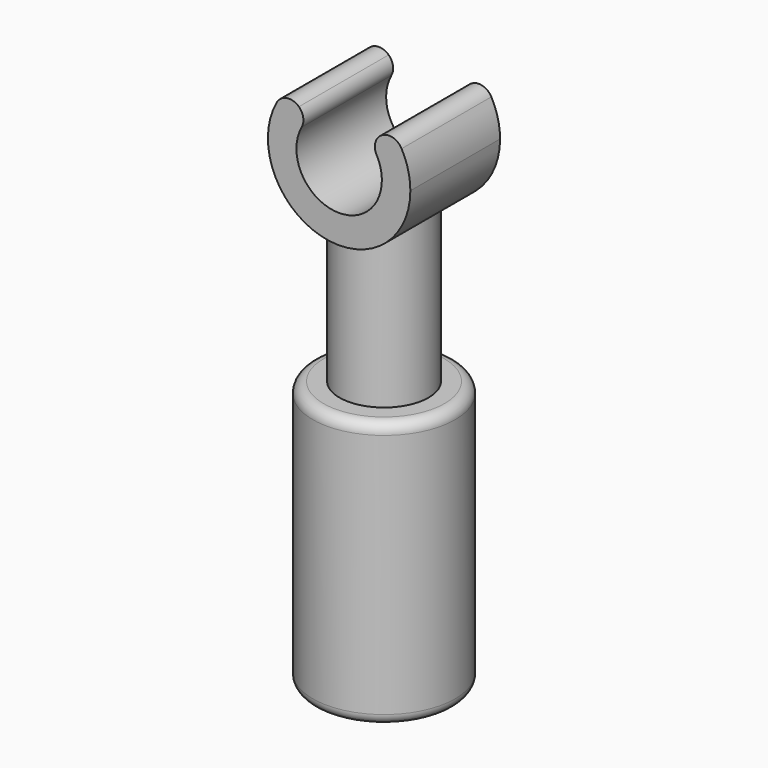
from build123d import *

# Parameters (mm, degrees)
F3_DEPTH = 3.15
F4_R     = 0.79999
F5_R     = 0.6


# Not quite as in the source:
# - a fillet or chamfer is up to 0.001 mm smaller than in the source, because OpenCascade refuses the exact size


with BuildPart() as f1:
    # F0 (on Front) → F1 (revolve)
    with BuildSketch(Plane.XZ):
        Polygon((0, 24.5), (0, 0), (4, 0), (4, 15), (2.5, 15), (2.5, 24.5), align=None)
    revolve(axis=Axis((0, 0, -0.3548332296), (0, 0, -1)))

    # F2 (on Front) → F3 (join, symmetric)
    with BuildSketch(Plane.XZ):
        with BuildLine():
            ThreePointArc((-2.9166666667, 29.7373446176), (-1.4719601444, 23.2806810659), (4, 27))
            ThreePointArc((4, 27), (3.7193189341, 28.4719601444), (2.9166666667, 29.7373446176))
            Line((2.9166666667, 29.7373446176), (1.75, 28.6424067706))
            ThreePointArc((1.75, 28.6424067706), (2.2315913604, 27.8831760866), (2.4, 27))
            ThreePointArc((2.4, 27), (-0.8831760866, 24.7684086396), (-1.75, 28.6424067706))
            Line((-1.75, 28.6424067706), (-2.9166666667, 29.7373446176))
        make_face()
    extrude(amount=F3_DEPTH, both=True)

    # F4 (radius 0.8 in the source; OpenCascade refuses exactly that, so slightly less here)
    f4_edges = [f1.edges().sort_by_distance(p)[0] for p in [
        (2.916667, -1.575, 29.737345),
        (2.916667, 1.575, 29.737345),
        (1.75, -1.575, 28.642407),
        (1.75, 1.575, 28.642407),
        (-1.75, 1.575, 28.642407),
        (-1.75, -1.575, 28.642407),
        (-2.916667, -1.575, 29.737345),
        (-2.916667, 1.575, 29.737345),
    ]]
    fillet(f4_edges, radius=F4_R)

    # F5
    f5_edges = [f1.edges().sort_by_distance(p)[0] for p in [
        (-4, 0, 0),
        (-4, 0, 15),
    ]]
    fillet(f5_edges, radius=F5_R)


solid = f1.part
